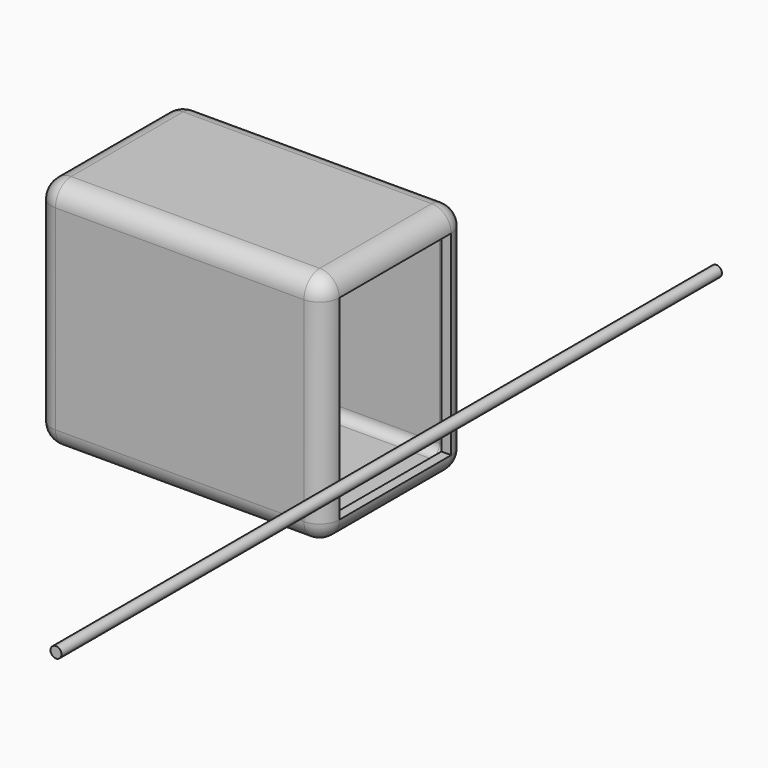
from build123d import *

# Parameters (mm, degrees)
F0_W     = 74.4587779045
F0_H     = 46.3549848646
F1_DEPTH = 60.706
F2_R     = 5.08
F3_T     = -2.54
F4_R     = 1.4228267919
F5_DEPTH = 213.614


# Not quite as in the source:
# - a shell that OpenCascade refuses in one call is made with other operations: the cavity is built on its own and cut out


with BuildPart() as f1:
    # F0 (on Top) → F1 (new body)
    with BuildSketch(Plane.XY):
        with Locations((-37.2293889523, -46.5841041878)):
            Rectangle(F0_W, F0_H)
    extrude(amount=F1_DEPTH)

    # F2
    f2_edges = [f1.edges().sort_by_distance(p)[0] for p in [
        (-37.229389, -23.406612, 60.706),
        (-74.458778, -46.584104, 60.706),
        (-37.229389, -69.761597, 60.706),
        (0, -46.584104, 60.706),
        (0, -69.761597, 30.353),
        (0, -23.406612, 30.353),
        (0, -46.584104, 0),
        (-74.458778, -69.761597, 30.353),
        (-37.229389, -69.761597, 0),
        (-74.458778, -23.406612, 30.353),
        (-74.458778, -46.584104, 0),
        (-37.229389, -23.406612, 0),
    ]]
    fillet(f2_edges, radius=F2_R)

    # F3: a shell. OpenCascade refuses it in one call, so the cavity is built on its own and cut out:
    # the body offset inwards by the wall thickness, plus a prism from it out through each open face.
    f3_core = offset(f1.part, amount=F3_T, mode=Mode.PRIVATE)
    f3_exits = [f3_core.faces().sort_by_distance(p)[0] for p in [
        (-2.54, -46.584104, 30.353),
        (-71.918778, -46.584104, 30.353),
    ]]
    add(f3_core, mode=Mode.SUBTRACT)
    extrude(f3_exits, amount=-F3_T, mode=Mode.SUBTRACT)


with BuildPart() as f5:
    # F4 (on Front) → F5 (new body)
    with BuildSketch(Plane.XZ):
        with Locations((45.8290316164, 50.3349490464)):
            Circle(F4_R)
    extrude(amount=F5_DEPTH)


solid = Compound([f1.part, f5.part])
